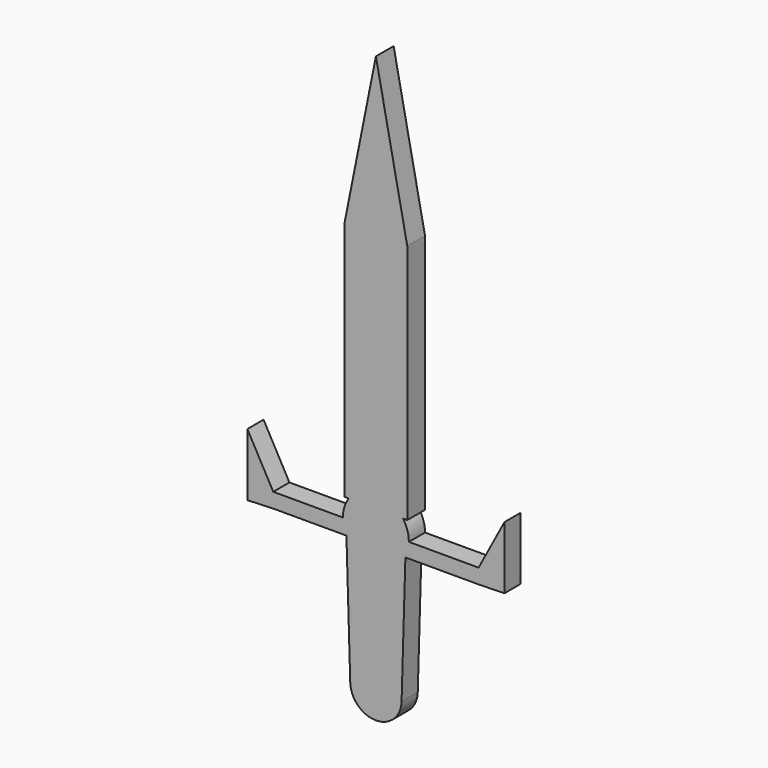
from build123d import *

# Parameters (mm, degrees)
F1_DEPTH = 5.05432
F2_W     = 15.6690403819
F2_H     = 21.0551657914
F3_DEPTH = 5.54634


# Not quite as in the source:
# - a feature names something its author has since deleted; it is built from what else it names


with BuildPart() as f1:
    # F0 (on Front) → F1 (new body)
    with BuildSketch(Plane.XZ):
        with BuildLine():
            ThreePointArc((-8.2431294521, 0), (-8.0211144228, -1.9002385587), (-7.3670285487, -3.6981175654))
            ThreePointArc((-7.3670285487, -3.6981175654), (0, -8.2431294521), (7.3670285487, -3.6981175654))
            ThreePointArc((7.3670285487, -3.6981175654), (8.0211144228, -1.9002385587), (8.2431294521, 0))
            Line((8.2431294521, 0), (0, 0))
            Line((0, 0), (-8.2431294521, 0))
        make_face()
        with BuildLine():
            Line((-25.6580412388, -3.6981175654), (-7.3670285487, -3.6981175654))
            ThreePointArc((-7.3670285487, -3.6981175654), (-8.0211144228, -1.9002385587), (-8.2431294521, 0))
            Line((-8.2431294521, 0), (-25.6580412388, 0))
            Line((-25.6580412388, 0), (-25.6580412388, -3.6981175654))
        make_face()
        with BuildLine():
            ThreePointArc((7.3670285487, -3.6981175654), (0, -8.2431294521), (-7.3670285487, -3.6981175654))
            Line((-7.3670285487, -3.6981175654), (-6.4152840294, -35.7396751265))
            ThreePointArc((-6.4152840294, -35.7396751265), (-0.0952885085, -29.131713029), (6.41811349, -35.5491191149))
            ThreePointArc((6.41811349, -35.5491191149), (6.4174060859, -35.6444076234), (6.4152840294, -35.7396751265))
            Line((6.4152840294, -35.7396751265), (7.3670285487, -3.6981175654))
        make_face()
        with BuildLine():
            ThreePointArc((8.2431294521, 0), (8.0211144228, -1.9002385587), (7.3670285487, -3.6981175654))
            Line((7.3670285487, -3.6981175654), (25.6736125353, -3.6981175654))
            Line((25.6736125353, -3.6981175654), (25.6736125353, 0))
            Line((25.6736125353, 0), (8.2431294521, 0))
        make_face()
        with BuildLine():
            ThreePointArc((8.2431294521, 0), (0, 8.2431294521), (-8.2431294521, 0))
            Line((-8.2431294521, 0), (0, 0))
            Line((0, 0), (8.2431294521, 0))
        make_face()
        Polygon((-32.1215167642, -3.9506237954), (-25.6580412388, -3.6981175654), (-25.6580412388, 0), (-32.1215167642, 11.7184091359), align=None)
        with BuildLine():
            ThreePointArc((6.41811349, -35.5491191149), (-0.0952885085, -29.131713029), (-6.4152840294, -35.7396751265))
            ThreePointArc((-6.4152840294, -35.7396751265), (0, -41.9672326049), (6.4152840294, -35.7396751265))
            ThreePointArc((6.4152840294, -35.7396751265), (6.4174060859, -35.6444076234), (6.41811349, -35.5491191149))
        make_face()
        Polygon((25.6736125353, 0), (25.6736125353, -3.6981175654), (32.1235085251, -3.5498465956), (32.1235085251, 12.1219534044), align=None)
    extrude(amount=-F1_DEPTH)

    # F2 (on Front) → F3 (join)
    with BuildSketch(Plane.XZ):
        Polygon((-7.834520191, 64.9923454344), (7.834520191, 64.9923454344), (0, 104.1657105088), align=None)
        with Locations((0, 54.4647625387)):
            Rectangle(F2_W, F2_H)
        Polygon((7.834520191, 4.6665664136), (7.834520191, 26.9957184792), (0, 26.9957184792), (-7.834520191, 26.9957184792), (-7.834520191, 4.6673454344), align=None)
        Polygon((7.834520191, 26.9957184792), (7.834520191, 43.937179643), (-7.834520191, 43.937179643), (-7.834520191, 26.9957184792), (0, 26.9957184792), align=None)
    extrude(amount=-F3_DEPTH)


solid = f1.part
